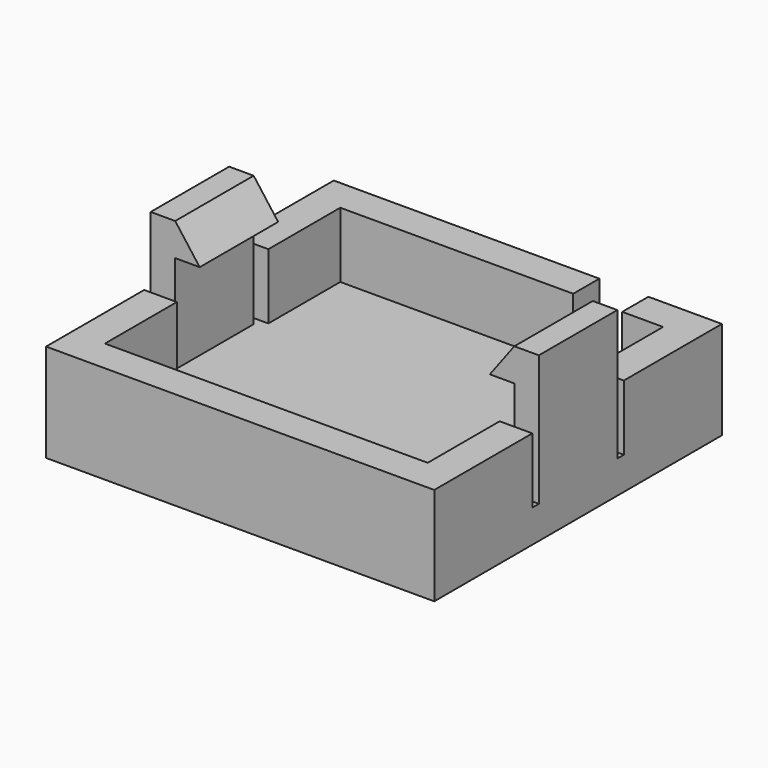
from build123d import *

# Parameters (mm, degrees)
F0_W      = 23.75
F0_H      = 22
F0_W_2    = 19.75
F0_H_2    = 18
F1_DEPTH  = 2
F2_DEPTH  = 6
F3_W      = 2
F3_H      = 0.5
F4_DEPTH  = 4
F5_DEPTH  = 4
F7_DEPTH  = 6
F8_W      = 3
F8_H      = 4
F9_DEPTH  = 5.2
F10_W     = 0.5
F10_H     = 6
F11_DEPTH = 8
F12_W     = 0.5
F12_H     = 6
F13_DEPTH = 8
F15_DEPTH = 6
F17_DEPTH = 6


# Not quite as in the source:
# - a feature names something its author has since deleted; it is built from what else it names


with BuildPart() as f1:
    # F0 (on Top) → F1 (new body)
    with BuildSketch(Plane.XY):
        Rectangle(F0_W, F0_H)
        Rectangle(F0_W_2, F0_H_2, mode=Mode.SUBTRACT)
        Rectangle(F0_W_2, F0_H_2)
    extrude(amount=F1_DEPTH)

    # F0 (on Top) → F2 (join)
    with BuildSketch(Plane.XY):
        Rectangle(F0_W, F0_H)
        Rectangle(F0_W_2, F0_H_2, mode=Mode.SUBTRACT)
    extrude(amount=F2_DEPTH)

    # F3 (on face) → F4 (cut)
    with BuildSketch(Plane.XY.offset(6)):
        Polygon((10.875, -3), (9.875, -3), (9.875, -3.5), (11.875, -3.5), (11.875, -3), align=None)
        Polygon((9.875, 3.5), (9.875, 3), (10.875, 3), (11.875, 3), (11.875, 3.5), align=None)
        with Locations((-10.875, 3.25)):
            Rectangle(F3_W, F3_H)
        with Locations((-10.875, -3.25)):
            Rectangle(F3_W, F3_H)
    extrude(amount=-F4_DEPTH, mode=Mode.SUBTRACT)

    # F5 (add): faces of the model
    f5_faces = [f1.faces().sort_by_distance(p)[0] for p in [
        (10.875, 0, 6),
        (-10.875, 0, 6),
    ]]
    extrude(f5_faces, amount=F5_DEPTH)

    # F6 (on face) → F7 (join)
    with BuildSketch(Plane.XZ.offset(3)):
        Polygon((11.875, 8), (11.875, 10), (10.375, 8), align=None)
    extrude(amount=-F7_DEPTH)

    # F8 (on face) → F9 (cut)
    with BuildSketch(Plane(origin=(0, 11, 0), x_dir=(-1, 0, 0), z_dir=(0, 1, 0))):
        with Locations((-5.875, 4)):
            Rectangle(F8_W, F8_H)
    extrude(amount=-F9_DEPTH, mode=Mode.SUBTRACT)

    # F10 (on face) → F11 (cut)
    with BuildSketch(Plane.XY.offset(10)):
        with Locations((-10.125, 0)):
            Rectangle(F10_W, F10_H)
    extrude(amount=-F11_DEPTH, mode=Mode.SUBTRACT)

    # F12 (on face) → F13 (cut)
    with BuildSketch(Plane.XY.offset(10)):
        with Locations((10.125, 0)):
            Rectangle(F12_W, F12_H)
    extrude(amount=-F13_DEPTH, mode=Mode.SUBTRACT)

    # F14 (on face) → F15 (join)
    with BuildSketch(Plane.XZ.offset(3)):
        Polygon((10.375, 8), (10.375, 10), (8.875, 8), align=None)
    extrude(amount=-F15_DEPTH)

    # F16 (on face) → F17 (join)
    with BuildSketch(Plane.XZ.offset(3)):
        Polygon((-8.875, 8), (-10.375, 10), (-10.375, 8), align=None)
    extrude(amount=-F17_DEPTH)


solid = f1.part
